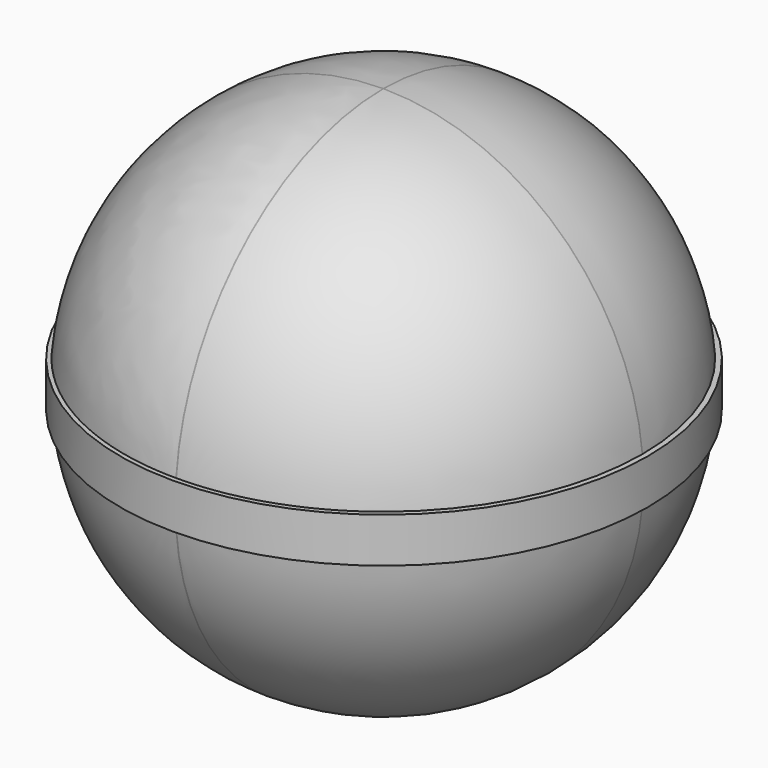
from build123d import *

# Parameters (mm, degrees)
F0_W         = 111.7644011974
F0_H         = 111.7644011974
F1_DEPTH     = 55.88
F2_R         = 55.8021322807
F3_R         = 55.8038
F5_T1_DEPTH  = 139.6679689167
F5_T3_DEPTH  = 0.1568011974
F5_T5_DEPTH  = 0.1524
F5_T7_DEPTH  = 139.6679689167
F5_T9_DEPTH  = 0.1568011974
F5_S13_W     = 56.919876
F5_S13_H     = 56.919876
F5_T14_DEPTH = 56.919876
F5_S19_W     = 56.919876
F5_S19_H     = 56.919876
F5_T20_DEPTH = 56.919876
F5_S25_W     = 56.919876
F5_S25_H     = 56.919876
F5_T26_DEPTH = 56.919876
F5_S31_W     = 56.919876
F5_S31_H     = 56.919876
F5_T32_DEPTH = 56.919876
F5_T36_ANGLE = 90
F5_T38_ANGLE = 90
F5_T40_ANGLE = 90
F5_T42_ANGLE = 90
F6_R         = 56.7270748454
F7_DEPTH     = 4.826


# Not quite as in the source:
# - a fillet or chamfer that OpenCascade refuses, or shapes differently, is made with other operations: its cross-section is extruded or revolved along the edge and cut away or added
# - a feature of the source that left no trace in its solid (it failed there, or was rolled back) is left out


with BuildPart() as f1:
    # F0 (on Front) → F1 (new body, symmetric)
    with BuildSketch(Plane.XZ):
        with Locations((-0.1386664808, 0)):
            Rectangle(F0_W, F0_H)
    extrude(amount=F1_DEPTH, both=True)

    # F2
    f2_edges = [f1.edges().sort_by_distance(p)[0] for p in [
        (-56.020867, 0, 55.882201),
    ]]
    fillet(f2_edges, radius=F2_R)

    # F3
    f3_edges = [f1.edges().sort_by_distance(p)[0] for p in [
        (55.743534, 0, 55.882201),
    ]]
    fillet(f3_edges, radius=F3_R)

    # F5: fillet of radius 55.8038 on 10 edges, made by hand

    # F5_s2 → F5_t1 (cut)
    with BuildSketch(Plane.YZ.offset(-139.7282347988)):
        with BuildLine():
            ThreePointArc((0.0762, 55.8822005987), (39.535445396, 39.5376459947), (55.88, 0.0784005987))
            Line((55.88, 0.0784005987), (56.996076, 0.0784005987))
            Line((56.996076, 0.0784005987), (56.996076, 56.9982765987))
            Line((56.996076, 56.9982765987), (0.0762, 56.9982765987))
            Line((0.0762, 56.9982765987), (0.0762, 55.8822005987))
        make_face()
        with BuildLine():
            ThreePointArc((-0.0762, 55.8822005987), (-39.535445396, 39.5376459947), (-55.88, 0.0784005987))
            Line((-55.88, 0.0784005987), (-56.996076, 0.0784005987))
            Line((-56.996076, 0.0784005987), (-56.996076, 56.9982765987))
            Line((-56.996076, 56.9982765987), (-0.0762, 56.9982765987))
            Line((-0.0762, 56.9982765987), (-0.0762, 55.8822005987))
        make_face()
    extrude(amount=F5_T1_DEPTH, mode=Mode.SUBTRACT)

    # F5_s4 → F5_t3 (cut)
    with BuildSketch(Plane.YZ.offset(-0.2170670795)):
        with BuildLine():
            ThreePointArc((55.88, -0.0784005987), (39.535445396, -39.5376459947), (0.0762, -55.8822005987))
            Line((0.0762, -55.8822005987), (0.0762, -56.9982765987))
            Line((0.0762, -56.9982765987), (56.996076, -56.9982765987))
            Line((56.996076, -56.9982765987), (56.996076, -0.0784005987))
            Line((56.996076, -0.0784005987), (55.88, -0.0784005987))
        make_face()
        with BuildLine():
            ThreePointArc((-55.88, -0.0784005987), (-39.535445396, -39.5376459947), (-0.0762, -55.8822005987))
            Line((-0.0762, -55.8822005987), (-0.0762, -56.9982765987))
            Line((-0.0762, -56.9982765987), (-56.996076, -56.9982765987))
            Line((-56.996076, -56.9982765987), (-56.996076, -0.0784005987))
            Line((-56.996076, -0.0784005987), (-55.88, -0.0784005987))
        make_face()
    extrude(amount=F5_T3_DEPTH, mode=Mode.SUBTRACT)

    # F5_s6 → F5_t5 (cut)
    with BuildSketch(Plane.XZ.offset(-0.0762)):
        with BuildLine():
            ThreePointArc((55.7435341179, -0.0784005987), (39.3989795139, -39.5376459947), (-0.0602658821, -55.8822005987))
            Line((-0.0602658821, -55.8822005987), (-0.0602658821, -56.9982765987))
            Line((-0.0602658821, -56.9982765987), (56.8596101179, -56.9982765987))
            Line((56.8596101179, -56.9982765987), (56.8596101179, -0.0784005987))
            Line((56.8596101179, -0.0784005987), (55.7435341179, -0.0784005987))
        make_face()
        with BuildLine():
            ThreePointArc((-56.0208670795, -0.0784005987), (-39.6763124755, -39.5376459947), (-0.2170670795, -55.8822005987))
            Line((-0.2170670795, -55.8822005987), (-0.2170670795, -56.9982765987))
            Line((-0.2170670795, -56.9982765987), (-57.1369430795, -56.9982765987))
            Line((-57.1369430795, -56.9982765987), (-57.1369430795, -0.0784005987))
            Line((-57.1369430795, -0.0784005987), (-56.0208670795, -0.0784005987))
        make_face()
    extrude(amount=F5_T5_DEPTH, mode=Mode.SUBTRACT)

    # F5_s8 → F5_t7 (cut)
    with BuildSketch(Plane.XY.offset(-0.0784005987)):
        with BuildLine():
            ThreePointArc((-0.2170670795, -55.88), (-39.6763124755, -39.535445396), (-56.0208670795, -0.0762))
            Line((-56.0208670795, -0.0762), (-57.1369430795, -0.0762))
            Line((-57.1369430795, -0.0762), (-57.1369430795, -56.996076))
            Line((-57.1369430795, -56.996076), (-0.2170670795, -56.996076))
            Line((-0.2170670795, -56.996076), (-0.2170670795, -55.88))
        make_face()
        with BuildLine():
            ThreePointArc((-0.2170670795, 55.88), (-39.6763124755, 39.535445396), (-56.0208670795, 0.0762))
            Line((-56.0208670795, 0.0762), (-57.1369430795, 0.0762))
            Line((-57.1369430795, 0.0762), (-57.1369430795, 56.996076))
            Line((-57.1369430795, 56.996076), (-0.2170670795, 56.996076))
            Line((-0.2170670795, 56.996076), (-0.2170670795, 55.88))
        make_face()
    extrude(amount=F5_T7_DEPTH, mode=Mode.SUBTRACT)

    # F5_s10 → F5_t9 (cut)
    with BuildSketch(Plane.XY.offset(-0.0784005987)):
        with BuildLine():
            ThreePointArc((-0.0602658821, -55.88), (39.3989795139, -39.535445396), (55.7435341179, -0.0762))
            Line((55.7435341179, -0.0762), (56.8596101179, -0.0762))
            Line((56.8596101179, -0.0762), (56.8596101179, -56.996076))
            Line((56.8596101179, -56.996076), (-0.0602658821, -56.996076))
            Line((-0.0602658821, -56.996076), (-0.0602658821, -55.88))
        make_face()
        with BuildLine():
            ThreePointArc((-0.0602658821, 55.88), (39.3989795139, 39.535445396), (55.7435341179, 0.0762))
            Line((55.7435341179, 0.0762), (56.8596101179, 0.0762))
            Line((56.8596101179, 0.0762), (56.8596101179, 56.996076))
            Line((56.8596101179, 56.996076), (-0.0602658821, 56.996076))
            Line((-0.0602658821, 56.996076), (-0.0602658821, 55.88))
        make_face()
    extrude(amount=F5_T9_DEPTH, mode=Mode.SUBTRACT)


with BuildPart() as f5_tool12:
    # F5_s13 → F5_t14 (new body)
    with BuildSketch(Plane.XZ.offset(-0.0762)):
        with Locations((-28.6770050795, -28.5383385987)):
            Rectangle(F5_S13_W, F5_S13_H)
    extrude(amount=-F5_T14_DEPTH)

    # F5_s15 → F5_t16 (revolve, cut)
    with BuildSketch(Plane(origin=(-0.2170670795, 0.0762, -0.0784005987), x_dir=(0.7071067812, 0, 0.7071067812), z_dir=(-0.7071067812, 0, 0.7071067812))):
        with BuildLine():
            ThreePointArc((0, -55.8038), (55.8038, 0), (0, 55.8038))
            Line((0, 55.8038), (0, -55.8038))
        make_face()
    revolve(axis=Axis((-0.2170670795, 0.0762, -0.0784005987), (0, 1, 0)), mode=Mode.SUBTRACT)


with BuildPart() as f1_1:
    add(f1.part)

    # F5_t11: cut F5_tool12
    add(f5_tool12.part, mode=Mode.SUBTRACT)


with BuildPart() as f5_tool18:
    # F5_s19 → F5_t20 (new body)
    with BuildSketch(Plane.XZ.offset(-0.0762)):
        with Locations((28.3996721179, -28.5383385987)):
            Rectangle(F5_S19_W, F5_S19_H)
    extrude(amount=-F5_T20_DEPTH)

    # F5_s21 → F5_t22 (revolve, cut)
    with BuildSketch(Plane(origin=(-0.0602658821, 0.0762, -0.0784005987), x_dir=(-0.7071067812, 0, 0.7071067812), z_dir=(-0.7071067812, 0, -0.7071067812))):
        with BuildLine():
            ThreePointArc((0, -55.8038), (55.8038, 0), (0, 55.8038))
            Line((0, 55.8038), (0, -55.8038))
        make_face()
    revolve(axis=Axis((-0.0602658821, 0.0762, -0.0784005987), (0, 1, 0)), mode=Mode.SUBTRACT)


with BuildPart() as f1_2:
    add(f1_1.part)

    # F5_t17: cut F5_tool18
    add(f5_tool18.part, mode=Mode.SUBTRACT)


with BuildPart() as f5_tool24:
    # F5_s25 → F5_t26 (new body)
    with BuildSketch(Plane.XZ.offset(0.0762)):
        with Locations((-28.6770050795, -28.5383385987)):
            Rectangle(F5_S25_W, F5_S25_H)
    extrude(amount=F5_T26_DEPTH)

    # F5_s27 → F5_t28 (revolve, cut)
    with BuildSketch(Plane(origin=(-0.2170670795, -0.0762, -0.0784005987), x_dir=(0.7071067812, 0, 0.7071067812), z_dir=(0.7071067812, 0, -0.7071067812))):
        with BuildLine():
            ThreePointArc((0, -55.8038), (55.8038, 0), (0, 55.8038))
            Line((0, 55.8038), (0, -55.8038))
        make_face()
    revolve(axis=Axis((-0.2170670795, -0.0762, -0.0784005987), (0, -1, 0)), mode=Mode.SUBTRACT)


with BuildPart() as f1_3:
    add(f1_2.part)

    # F5_t23: cut F5_tool24
    add(f5_tool24.part, mode=Mode.SUBTRACT)


with BuildPart() as f5_tool30:
    # F5_s31 → F5_t32 (new body)
    with BuildSketch(Plane.XZ.offset(0.0762)):
        with Locations((28.3996721179, -28.5383385987)):
            Rectangle(F5_S31_W, F5_S31_H)
    extrude(amount=F5_T32_DEPTH)

    # F5_s33 → F5_t34 (revolve, cut)
    with BuildSketch(Plane(origin=(-0.0602658821, -0.0762, -0.0784005987), x_dir=(-0.7071067812, 0, 0.7071067812), z_dir=(0.7071067812, 0, 0.7071067812))):
        with BuildLine():
            ThreePointArc((0, -55.8038), (55.8038, 0), (0, 55.8038))
            Line((0, 55.8038), (0, -55.8038))
        make_face()
    revolve(axis=Axis((-0.0602658821, -0.0762, -0.0784005987), (0, -1, 0)), mode=Mode.SUBTRACT)


with BuildPart() as f1_4:
    add(f1_3.part)

    # F5_t29: cut F5_tool30
    add(f5_tool30.part, mode=Mode.SUBTRACT)

    # F5_s35 → F5_t36 (revolve, cut)
    with BuildSketch(Plane.YZ.offset(-0.0602658821)):
        with BuildLine():
            ThreePointArc((55.88, 0.0784005987), (39.535445396, 39.5376459947), (0.0762, 55.8822005987))
            Line((0.0762, 55.8822005987), (0.0762, 56.9982765987))
            Line((0.0762, 56.9982765987), (56.996076, 56.9982765987))
            Line((56.996076, 56.9982765987), (56.996076, 0.0784005987))
            Line((56.996076, 0.0784005987), (55.88, 0.0784005987))
        make_face()
    revolve(axis=Axis((-0.0602658821, 55.88, 0.0784005987), (0, 1, 0)), revolution_arc=F5_T36_ANGLE, mode=Mode.SUBTRACT)

    # F5_s37 → F5_t38 (revolve, cut)
    with BuildSketch(Plane.YZ.offset(-0.2187347988)):
        with BuildLine():
            ThreePointArc((55.8799999751, 0.080068318), (39.5348557638, 39.5382356181), (0.0762, 55.8822005987))
            Line((0.0762, 55.8822005987), (0.0762, 56.9982765987))
            Line((0.0762, 56.9982765987), (56.996076, 56.9982765987))
            Line((56.996076, 56.9982765987), (56.996076, 0.080068318))
            Line((56.996076, 0.080068318), (55.8799999751, 0.080068318))
        make_face()
    revolve(axis=Axis((-0.2187347988, 55.88, 0.080068318), (0, -1, 0)), revolution_arc=F5_T38_ANGLE, mode=Mode.SUBTRACT)

    # F5_s39 → F5_t40 (revolve, cut)
    with BuildSketch(Plane.YZ.offset(-0.0602658821)):
        with BuildLine():
            ThreePointArc((-0.0762, 55.8822005987), (-39.535445396, 39.5376459947), (-55.88, 0.0784005987))
            Line((-55.88, 0.0784005987), (-56.996076, 0.0784005987))
            Line((-56.996076, 0.0784005987), (-56.996076, 56.9982765987))
            Line((-56.996076, 56.9982765987), (-0.0762, 56.9982765987))
            Line((-0.0762, 56.9982765987), (-0.0762, 55.8822005987))
        make_face()
    revolve(axis=Axis((-0.0602658821, -55.88, 0.0784005987), (0, 1, 0)), revolution_arc=F5_T40_ANGLE, mode=Mode.SUBTRACT)

    # F5_s41 → F5_t42 (revolve, cut)
    with BuildSketch(Plane.YZ.offset(-0.2187347988)):
        with BuildLine():
            ThreePointArc((-0.0762, 55.8822005987), (-39.5348557638, 39.5382356181), (-55.8799999751, 0.080068318))
            Line((-55.8799999751, 0.080068318), (-56.996076, 0.080068318))
            Line((-56.996076, 0.080068318), (-56.996076, 56.9982765987))
            Line((-56.996076, 56.9982765987), (-0.0762, 56.9982765987))
            Line((-0.0762, 56.9982765987), (-0.0762, 55.8822005987))
        make_face()
    revolve(axis=Axis((-0.2187347988, -55.88, 0.080068318), (0, -1, 0)), revolution_arc=F5_T42_ANGLE, mode=Mode.SUBTRACT)

    # F6 (on Top) → F7 (join, symmetric)
    with BuildSketch(Plane.XY):
        Circle(F6_R)
    extrude(amount=F7_DEPTH, both=True)


solid = f1_4.part
